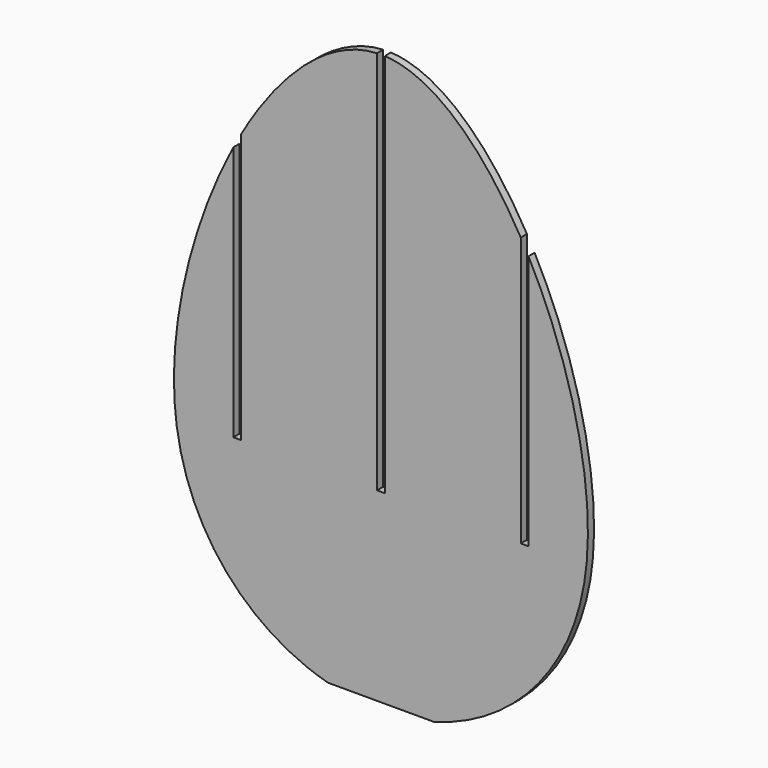
from build123d import *

# Parameters (mm, degrees)
F1_DEPTH = 3


# Not quite as in the source:
# - a feature names something its author has since deleted; it is built from what else it names


with BuildPart() as f1:
    # F0 (on Front) → F1 (new body)
    with BuildSketch(Plane.XZ):
        with BuildLine():
            Line((-95.6991912493, -140.1659290001), (-95.6991912493, 9.7979199733))
            add(Edge.make_bspline(
                [(-95.6991912493, 9.7979199733), (-114.9403248651, 8.8727934734), (-134.0676037648, -9.7150772734), (-148.6991912496, -35.2231978093)],
                knots=[0.0032045269, 0.0032045269, 0.0032045269, 0.0032045269, 0.1265346274, 0.1265346274, 0.1265346274, 0.1265346274], degree=3))
            Line((-148.6991912496, -35.2231978093), (-148.6991912415, -140.1659290001))
            Line((-148.6991912415, -140.1659290001), (-151.6991912415, -140.1659290001))
            Line((-151.6991912415, -140.1659290001), (-151.6991912492, -40.6684138407))
            add(Edge.make_bspline(
                [(-151.6991912492, -40.6684138407), (-167.8134864464, -71.1210787155), (-189.9683027369, -159.0658708259), (-144.3602498784, -204.2889070632), (-114.8366912492, -212.3738275092)],
                knots=[0.135152904, 0.135152904, 0.135152904, 0.135152904, 0.2772924741, 0.4585993514, 0.4585993514, 0.4585993514, 0.4585993514], degree=3))
            Line((-114.8366912492, -212.3738275092), (-73.5616912492, -212.3738275092))
            add(Edge.make_bspline(
                [(-73.5616912492, -212.3738275092), (-44.03813262, -204.2889070632), (1.5699202449, -159.0658708196), (-20.5848960581, -71.1210786912), (-36.6991912644, -40.6684138119)],
                knots=[0.5414006486, 0.5414006486, 0.5414006486, 0.5414006486, 0.7227075259, 0.8648470961, 0.8648470961, 0.8648470961, 0.8648470961], degree=3))
            Line((-36.6991912644, -40.6684138119), (-36.6991912645, -140.1659290001))
            Line((-36.6991912645, -140.1659290001), (-39.6991912645, -140.1659290001))
            Line((-39.6991912645, -140.1659290001), (-39.6991912644, -35.223197782))
            add(Edge.make_bspline(
                [(-39.6991912644, -35.223197782), (-54.3307787472, -9.71507726), (-73.4580576403, 8.8727934739), (-92.6991912493, 9.7979199734)],
                knots=[0.8734653727, 0.8734653727, 0.8734653727, 0.8734653727, 0.9967954731, 0.9967954731, 0.9967954731, 0.9967954731], degree=3))
            Line((-92.6991912493, 9.7979199734), (-92.6991912493, -140.1659290001))
            Line((-92.6991912493, -140.1659290001), (-95.6991912493, -140.1659290001))
        make_face()
    extrude(amount=F1_DEPTH)


solid = f1.part
